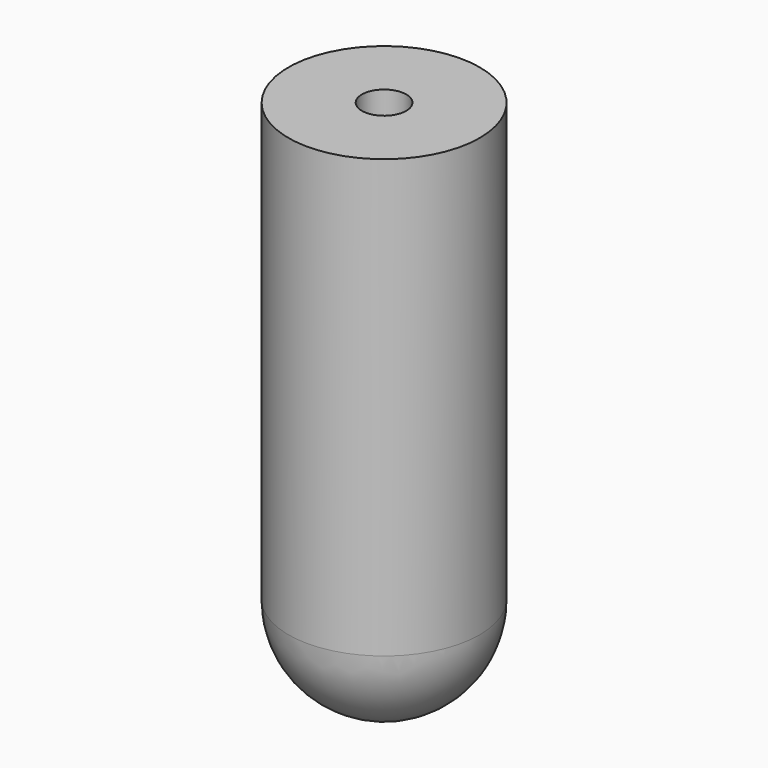
from build123d import *

# Parameters (mm, degrees)
F0_R     = 14
F1_DEPTH = 64
F6_R     = 3.25
F7_DEPTH = 69.14147


# Not quite as in the source:
# - a feature of the source that left no trace in its solid (it failed there, or was rolled back) is left out


with BuildPart() as f1:
    # F0 (on Top) → F1 (new body)
    with BuildSketch(Plane.XY):
        Circle(F0_R)
    extrude(amount=F1_DEPTH)

    # F2 (on Front) → F3 (revolve)
    with BuildSketch(Plane.XZ):
        with BuildLine():
            Line((0, 0), (-14, 0))
            ThreePointArc((-14, 0), (0, -14), (14, 0))
            Line((14, 0), (0, 0))
        make_face()
    revolve(axis=Axis((0, 0, 0), (1, 0, 0)))

    # F6 (on offset) → F7 (cut)
    with BuildSketch(Plane.XY.offset(-5)):
        Circle(F6_R)
    extrude(amount=F7_DEPTH, mode=Mode.SUBTRACT)


solid = f1.part
